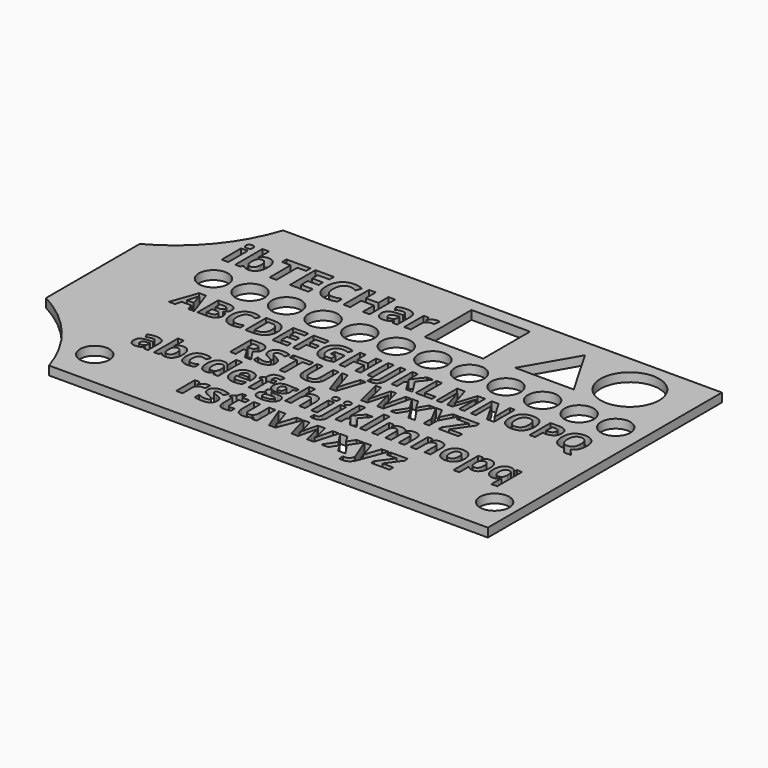
from build123d import *

# Parameters (mm, degrees)
F1_DEPTH       = 3
F2_W           = 20
F2_H           = 20
F2_R           = 10
F2_R_2         = 5
F2_TEXT_SIZE   = 15.2791514614
F2_TEXT_SIZE_2 = 12.4876308344
F2_TEXT_SIZE_3 = 12.6310595781
F2_TEXT_SIZE_4 = 13.4983857099
F2_TEXT_SIZE_5 = 14.5998722511
F3_DEPTH       = 25


# Not quite as in the source:
# - Text() gives the source's letters only with a copy of the font that has no kerning and outlines rounded to 1/6400 em; it was checked with that copy


with BuildPart() as f1:
    # F0 (on Top) → F1 (new body)
    with BuildSketch(Plane.XY):
        with BuildLine():
            Line((-62.5, -50), (87.5, -50))
            Line((87.5, -50), (87.5, 50))
            Line((87.5, 50), (-62.5, 50))
            ThreePointArc((-62.5, 50), (-72.0768540724, 32.5640450603), (-87.5, 20))
            Line((-87.5, 20), (-87.5, -20))
            ThreePointArc((-87.5, -20), (-72.0768540724, -32.5640450603), (-62.5, -50))
        make_face()
    extrude(amount=F1_DEPTH)

    # F2 (on face) → F3 (cut)
    with BuildSketch(Plane.XY.offset(3)):
        with Locations((15.5, 35.5)):
            Rectangle(F2_W, F2_H)
        Polygon((45.5, 44), (35.5, 26.6794919243), (55.5, 26.6794919243), align=None)
        with Locations((67.2527924006, 36)):
            Circle(F2_R)
        with Locations((-59.556286782, 16.5726331281)):
            Circle(F2_R_2)
        with Locations((-47.056286782, 16.5726331281)):
            Circle(F2_R_2)
        with Locations((-34.556286782, 16.5726331281)):
            Circle(F2_R_2)
        with Locations((-22.056286782, 16.5726331281)):
            Circle(F2_R_2)
        with Locations((-9.556286782, 16.5726331281)):
            Circle(F2_R_2)
        with Locations((2.943713218, 16.5726331281)):
            Circle(F2_R_2)
        with Locations((15.443713218, 16.5726331281)):
            Circle(F2_R_2)
        with Locations((27.943713218, 16.5726331281)):
            Circle(F2_R_2)
        with Locations((40.443713218, 16.5726331281)):
            Circle(F2_R_2)
        with Locations((52.943713218, 16.5726331281)):
            Circle(F2_R_2)
        with Locations((65.443713218, 16.5726331281)):
            Circle(F2_R_2)
        with Locations((77.943713218, 16.5726331281)):
            Circle(F2_R_2)
        with Locations((79.7107368708, -37.375087738)):
            Circle(F2_R_2)
        with Locations((-56.9626055658, -37.375087738)):
            Circle(F2_R_2)
        with Locations((-65.9527933431, 26.5710618959)):
            Text('ibTECHar', F2_TEXT_SIZE, font='Open Sans', font_style=FontStyle.BOLD, text_align=(TextAlign.LEFT, TextAlign.BOTTOM))
        with Locations((-60.4890270019, -1.2526484364)):
            Text('ABCDEFGHIJKLMNOPQ', F2_TEXT_SIZE_2, font='Open Sans', font_style=FontStyle.BOLD, text_align=(TextAlign.LEFT, TextAlign.BOTTOM))
        with Locations((-30.821820721, -13.654621024)):
            Text('RSTUV WXYZ', F2_TEXT_SIZE_3, font='Open Sans', font_style=FontStyle.BOLD, text_align=(TextAlign.LEFT, TextAlign.BOTTOM))
        with Locations((-54.6025000513, -26.5329735457)):
            Text('abcdefghijklmnopq', F2_TEXT_SIZE_4, font='Open Sans', font_style=FontStyle.BOLD, text_align=(TextAlign.LEFT, TextAlign.BOTTOM))
        with Locations((-27.9626809061, -40.2714257799)):
            Text('rstuvwxyz', F2_TEXT_SIZE_5, font='Open Sans', font_style=FontStyle.BOLD, text_align=(TextAlign.LEFT, TextAlign.BOTTOM))
    extrude(amount=-F3_DEPTH, mode=Mode.SUBTRACT)


solid = f1.part
